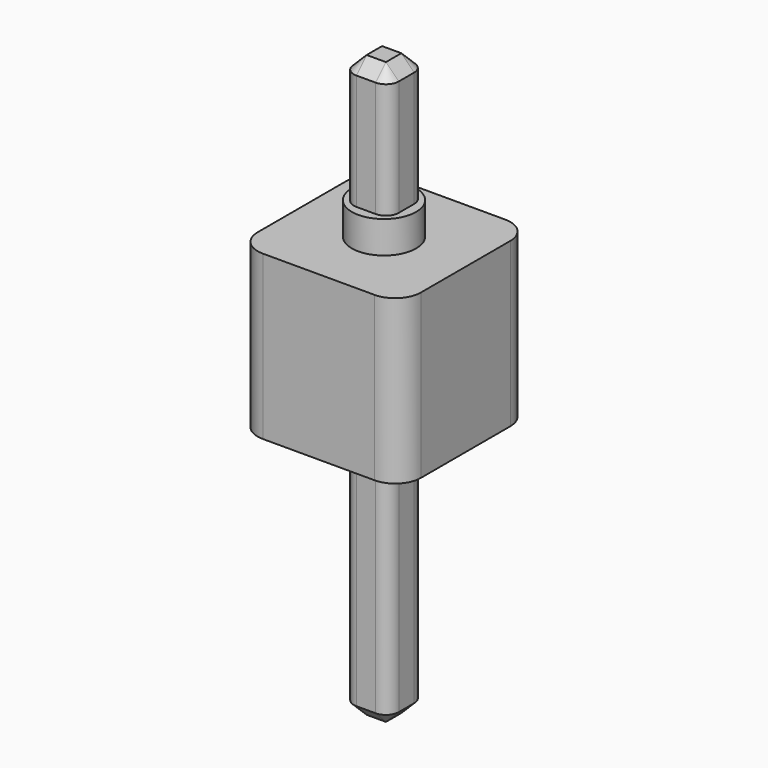
from build123d import *

# Parameters (mm, degrees)
F1_DEPTH = 2.54
F2_R     = 0.5
F3_DEPTH = 0.5
F5_DEPTH = 2
F6_SIZE  = 0.2
F8_DEPTH = 4
F9_SIZE  = 0.19999


# Not quite as in the source:
# - a fillet or chamfer is up to 0.001 mm smaller than in the source, because OpenCascade refuses the exact size


with BuildPart() as f1:
    # F0 (on Top) → F1 (new body)
    with BuildSketch(Plane.XY):
        with BuildLine():
            Line((-0.87, -1.27), (0.87, -1.27))
            ThreePointArc((0.87, -1.27), (1.1528427125, -1.1528427125), (1.27, -0.87))
            Line((1.27, -0.87), (1.27, 0.87))
            ThreePointArc((1.27, 0.87), (1.1528427125, 1.1528427125), (0.87, 1.27))
            Line((0.87, 1.27), (-0.87, 1.27))
            ThreePointArc((-0.87, 1.27), (-1.1528427125, 1.1528427125), (-1.27, 0.87))
            Line((-1.27, 0.87), (-1.27, -0.87))
            ThreePointArc((-1.27, -0.87), (-1.1528427125, -1.1528427125), (-0.87, -1.27))
        make_face()
    extrude(amount=F1_DEPTH)

    # F2 (on face) → F3 (join)
    with BuildSketch(Plane.XY.offset(2.54)):
        Circle(F2_R)
    extrude(amount=F3_DEPTH)


with BuildPart() as f5:
    # F4 (on face) → F5 (new body)
    with BuildSketch(Plane.XY.offset(3.04)):
        with BuildLine():
            Line((0.15, 0.35), (-0.15, 0.35))
            ThreePointArc((-0.15, 0.35), (-0.2914213562, 0.2914213562), (-0.35, 0.15))
            Line((-0.35, 0.15), (-0.35, -0.15))
            ThreePointArc((-0.35, -0.15), (-0.2914213562, -0.2914213562), (-0.15, -0.35))
            Line((-0.15, -0.35), (0.15, -0.35))
            ThreePointArc((0.15, -0.35), (0.2914213562, -0.2914213562), (0.35, -0.15))
            Line((0.35, -0.15), (0.35, 0.15))
            ThreePointArc((0.35, 0.15), (0.2914213562, 0.2914213562), (0.15, 0.35))
        make_face()
    extrude(amount=F5_DEPTH)

    # F6
    f6_edges = [f5.edges().sort_by_distance(p)[0] for p in [
        (0.35, 0, 5.04),
        (0.291421, 0.291421, 5.04),
        (0, 0.35, 5.04),
        (-0.291421, 0.291421, 5.04),
        (-0.35, 0, 5.04),
        (-0.291421, -0.291421, 5.04),
        (0, -0.35, 5.04),
        (0.291421, -0.291421, 5.04),
    ]]
    chamfer(f6_edges, length=F6_SIZE)


with BuildPart() as f8:
    # F7 (on face) → F8 (new body)
    with BuildSketch(Plane(origin=(0, 0, 0), x_dir=(1, 0, 0), z_dir=(0, 0, -1))):
        with BuildLine():
            ThreePointArc((-0.35, -0.15), (-0.2914213562, -0.2914213562), (-0.15, -0.35))
            Line((-0.15, -0.35), (0.15, -0.35))
            ThreePointArc((0.15, -0.35), (0.2914213562, -0.2914213562), (0.35, -0.15))
            Line((0.35, -0.15), (0.35, 0.15))
            ThreePointArc((0.35, 0.15), (0.2914213562, 0.2914213562), (0.15, 0.35))
            Line((0.15, 0.35), (-0.15, 0.35))
            ThreePointArc((-0.15, 0.35), (-0.2914213562, 0.2914213562), (-0.35, 0.15))
            Line((-0.35, 0.15), (-0.35, -0.15))
        make_face()
    extrude(amount=F8_DEPTH)

    # F9 (size 0.2 in the source; OpenCascade refuses exactly that, so slightly less here)
    f9_edges = [f8.edges().sort_by_distance(p)[0] for p in [
        (-0.291421, 0.291421, -4),
        (0, 0.35, -4),
        (0.291421, 0.291421, -4),
        (0.35, 0, -4),
        (0.291421, -0.291421, -4),
        (0, -0.35, -4),
        (-0.291421, -0.291421, -4),
        (-0.35, 0, -4),
    ]]
    chamfer(f9_edges, length=F9_SIZE)


solid = Compound([f1.part, f5.part, f8.part])
